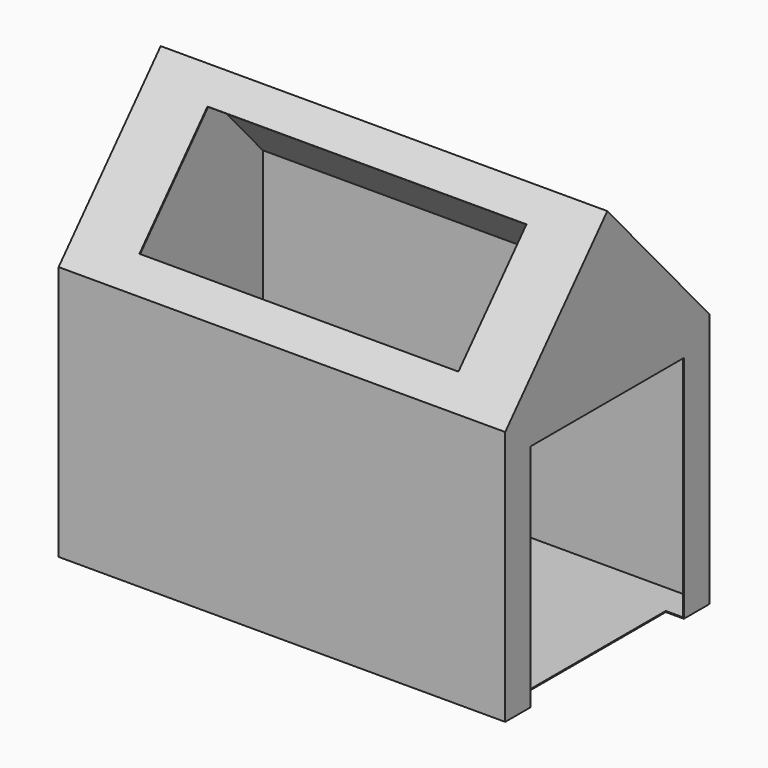
from build123d import *

# Parameters (mm, degrees)
F0_W         = 1066.8
F0_H         = 609.6
F1_DEPTH     = 609.6
F2_T         = -2.54
F3_W         = 457.2
F3_H         = 548.64
F4_DEPTH     = 43.18
F6_DEPTH     = 1066.8
F7_T         = 2.54
F7_T3_DEPTH  = 7.62
F7_T5_DEPTH  = 7.62
F7_T7_DEPTH  = 612.14
F7_T9_DEPTH  = 78.74
F7_T11_DEPTH = 78.74
F7_T13_DEPTH = 1066.8
F7_T15_DEPTH = 609.6
F8_W         = 762
F8_H         = 304.8
F9_DEPTH     = 25.4


# Not quite as in the source:
# - a shell that OpenCascade refuses in one call is made with other operations: the cavity is built on its own and cut out


with BuildPart() as f1:
    # F0 (on Front) → F1 (new body)
    with BuildSketch(Plane.XZ):
        with Locations((533.4, -304.8)):
            Rectangle(F0_W, F0_H)
    extrude(amount=F1_DEPTH)

    # F2
    f2_openings = [f1.faces().sort_by_distance(p)[0] for p in [
        (533.4, -304.8, 0),
    ]]
    offset(amount=F2_T, openings=f2_openings)

    # F3 (on face) → F4 (cut)
    with BuildSketch(Plane.YZ.offset(1066.8)):
        with Locations((-304.8, -335.28)):
            Rectangle(F3_W, F3_H)
    extrude(amount=-F4_DEPTH, mode=Mode.SUBTRACT)

    # F5 (on face) → F6 (join)
    with BuildSketch(Plane(origin=(0, 0, 0), x_dir=(0, -1, 0), z_dir=(-1, 0, 0))):
        Polygon((304.8, 340.776759771), (0, 0), (609.6, 0), align=None)
    extrude(amount=-F6_DEPTH)

    # F7: shell of thickness 2.54, made by hand


with BuildPart() as f7_core1:
    # F7_t2: copy of F1
    add(f1.part)

    # the walls: a layer under each face that stays
    f7_faces = [f7_core1.faces().sort_by_distance(p)[0] for p in [
        (0, -304.8, -134.4116201145),
        (533.4, -304.8, -609.6),
        (533.4, 0, -304.8),
        (533.4, -609.6, -304.8),
        (533.4, -152.4, 170.3883798855),
        (533.4, -457.2, 170.3883798855),
        (1066.8, -304.8, 182.3806331425),
        (1065.3606666667, -76.2, -591.312),
        (1023.62, -304.8, -608.33),
        (1065.3606666667, -533.4, -79.248),
        (1065.53, -304.8, -60.96),
        (1064.26, -563.88, -563.6985714286),
        (533.4, -304.8, -607.06),
        (533.4, -607.06, -303.53),
        (533.4, -2.54, -303.53),
        (2.54, -304.8, -303.53),
    ]]
    thicken(f7_faces, amount=-F7_T, mode=Mode.SUBTRACT)

    # F7_s4 → F7_t3 (cut)
    with BuildSketch(Plane.YZ.offset(1061.72)):
        Polygon((-76.2254, -60.9854), (-73.66, -60.96), (-73.66, -58.42), (-76.2, -58.42), align=None)
        Polygon((-533.3746, -60.9854), (-535.94, -60.96), (-535.94, -58.42), (-533.4, -58.42), align=None)
    extrude(amount=F7_T3_DEPTH, mode=Mode.SUBTRACT)

    # F7_s6 → F7_t5 (cut)
    with BuildSketch(Plane.XY.offset(-612.14)):
        Polygon((1023.6454, -76.2254), (1023.62, -73.66), (1021.08, -73.66), (1021.08, -76.2), align=None)
        Polygon((1023.6454, -533.3746), (1021.08, -533.4), (1021.08, -535.94), (1023.62, -535.94), align=None)
    extrude(amount=F7_T5_DEPTH, mode=Mode.SUBTRACT)

    # F7_s8 → F7_t7 (cut)
    with BuildSketch(Plane.XY.offset(-609.6)):
        Polygon((1064.2346, -607.0346), (1066.8, -607.06), (1066.8, -609.6), (1064.26, -609.6), align=None)
        Polygon((1064.2346, -2.5654), (1066.8, -2.54), (1066.8, 0), (1064.26, 0), align=None)
        Polygon((2.5654, -607.0346), (2.54, -609.6), (0, -609.6), (0, -607.06), align=None)
        Polygon((2.5654, -2.5654), (2.54, 0), (0, 0), (0, -2.54), align=None)
    extrude(amount=F7_T7_DEPTH, mode=Mode.SUBTRACT)

    # F7_s10 → F7_t9 (cut)
    with BuildSketch(Plane.XZ.offset(530.86)):
        Polygon((1064.2346, -607.0346), (1066.8, -607.06), (1066.8, -609.6), (1064.26, -609.6), align=None)
    extrude(amount=F7_T9_DEPTH, mode=Mode.SUBTRACT)

    # F7_s12 → F7_t11 (cut)
    with BuildSketch(Plane.XZ):
        Polygon((1064.2346, -607.0346), (1066.8, -607.06), (1066.8, -609.6), (1064.26, -609.6), align=None)
    extrude(amount=F7_T11_DEPTH, mode=Mode.SUBTRACT)

    # F7_s14 → F7_t13 (cut)
    with BuildSketch(Plane.YZ):
        Polygon((-607.0346, -607.0346), (-607.06, -609.6), (-609.6, -609.6), (-609.6, -607.06), align=None)
        Polygon((-2.5654, -607.0346), (-2.54, -609.6), (0, -609.6), (0, -607.06), align=None)
    extrude(amount=F7_T13_DEPTH, mode=Mode.SUBTRACT)

    # F7_s16 → F7_t15 (cut)
    with BuildSketch(Plane.XZ):
        Polygon((2.5654, -607.0346), (2.54, -609.6), (0, -609.6), (0, -607.06), align=None)
    extrude(amount=F7_T15_DEPTH, mode=Mode.SUBTRACT)


with BuildPart() as f1_1:
    add(f1.part)

    # what is left inside the walls is the cavity
    f7_cavity = [f7_core1.part.solids().sort_by_distance(p)[0] for p in [
        (710.353333, -304.8, 0.0254),
    ]]
    add(f7_cavity, mode=Mode.SUBTRACT)

    # F8 (on face) → F9 (cut)
    with BuildSketch(Plane(origin=(0, -338.6666666667, 302.912675352), x_dir=(1, 0, 0), z_dir=(0, -0.7453559925, 0.6666666667))):
        with Locations((533.4, -177.8)):
            Rectangle(F8_W, F8_H)
    extrude(amount=-F9_DEPTH, mode=Mode.SUBTRACT)


solid = f1_1.part
